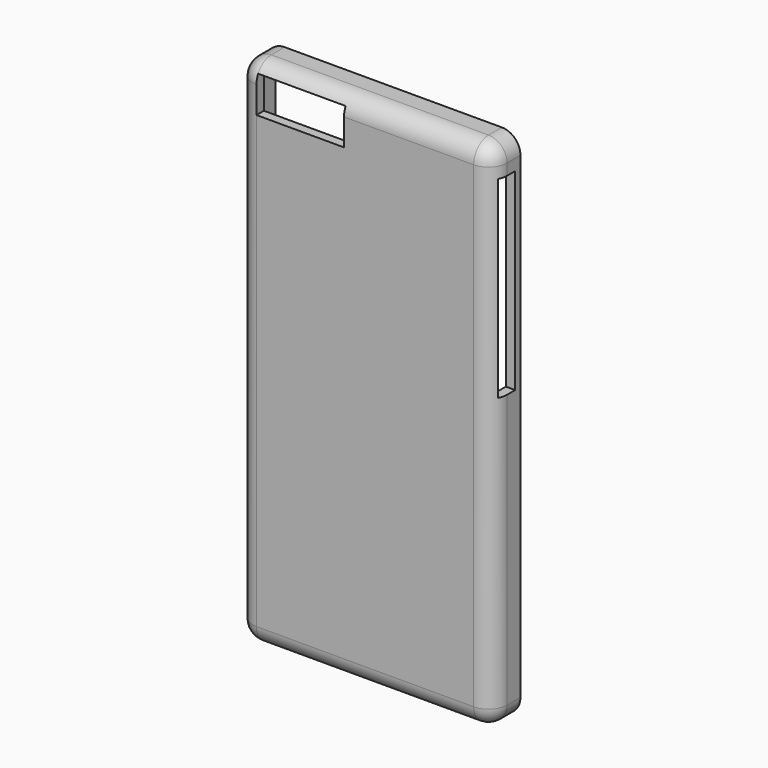
from build123d import *

# Parameters (mm, degrees)
F0_W        = 69.596
F0_H        = 140.716
F1_DEPTH    = 9.652
F2_R        = 5.08
F3_T1_DEPTH = 17.272
F3_S5_W     = 5.08
F3_S5_H     = 5.08
F3_T6_DEPTH = 5.08
F4_T1_DEPTH = 17.272
F4_S5_W     = 5.08
F4_S5_H     = 5.08
F4_T6_DEPTH = 5.08
F5_T1_DEPTH = 17.272
F5_S5_W     = 5.08
F5_S5_H     = 5.08
F5_T6_DEPTH = 5.08
F6_T        = -2.54
F7_W        = 23.9500291884
F7_H        = 9.7231566906
F8_DEPTH    = 25.4
F9_W        = 5.1087748725
F9_H        = 52.7357356623
F10_DEPTH   = 25.4
F11_W       = 4.6143759973
F11_H       = 14.0079259872
F12_DEPTH   = 25.4
F14_W       = 56.6909182817
F14_H       = 3.6255817395
F15_DEPTH   = 25.4


# Not quite as in the source:
# - a fillet or chamfer that OpenCascade refuses, or shapes differently, is made with other operations: its cross-section is extruded or revolved along the edge and cut away or added


with BuildPart() as f1:
    # F0 (on Front) → F1 (new body)
    with BuildSketch(Plane.XZ):
        Rectangle(F0_W, F0_H)
    extrude(amount=F1_DEPTH)

    # F2
    f2_edges = [f1.edges().sort_by_distance(p)[0] for p in [
        (-34.798, -4.826, 70.358),
        (0, -9.652, 70.358),
        (-34.798, -9.652, 0),
        (0, -9.652, -70.358),
        (34.798, -9.652, 0),
    ]]
    fillet(f2_edges, radius=F2_R)

    # F3: fillet of radius 5.08 on 1 edges, made by hand

    # F3_s2 → F3_t1 (cut)
    with BuildSketch(Plane.XZ.offset(-12.7)):
        with BuildLine():
            ThreePointArc((29.718, 70.358), (33.3101024484, 68.8701024484), (34.798, 65.278))
            Line((34.798, 65.278), (34.798, 70.358))
            Line((34.798, 70.358), (29.718, 70.358))
        make_face()
    extrude(amount=F3_T1_DEPTH, mode=Mode.SUBTRACT)


with BuildPart() as f3_tool4:
    # F3_s5 → F3_t6 (new body)
    with BuildSketch(Plane.XY.offset(65.278)):
        with Locations((32.258, -7.112)):
            Rectangle(F3_S5_W, F3_S5_H)
    extrude(amount=F3_T6_DEPTH)

    # F3_s7 → F3_t8 (revolve, cut)
    with BuildSketch(Plane(origin=(29.718, -4.572, 65.278), x_dir=(-0.7071067812, 0.7071067812, 0), z_dir=(0.7071067812, 0.7071067812, 0))):
        with BuildLine():
            ThreePointArc((0, -5.08), (5.08, 0), (0, 5.08))
            Line((0, 5.08), (0, -5.08))
        make_face()
    revolve(axis=Axis((29.718, -4.572, 65.278), (0, 0, 1)), mode=Mode.SUBTRACT)


with BuildPart() as f1_1:
    add(f1.part)

    # F3_t3: cut F3_tool4
    add(f3_tool4.part, mode=Mode.SUBTRACT)

    # F4: fillet of radius 5.08 on 1 edges, made by hand

    # F4_s2 → F4_t1 (cut)
    with BuildSketch(Plane.XZ.offset(-12.7)):
        with BuildLine():
            ThreePointArc((-29.718, -70.358), (-33.3101024484, -68.8701024484), (-34.798, -65.278))
            Line((-34.798, -65.278), (-34.798, -70.358))
            Line((-34.798, -70.358), (-29.718, -70.358))
        make_face()
    extrude(amount=F4_T1_DEPTH, mode=Mode.SUBTRACT)


with BuildPart() as f4_tool4:
    # F4_s5 → F4_t6 (new body)
    with BuildSketch(Plane.XY.offset(-65.278)):
        with Locations((-32.258, -7.112)):
            Rectangle(F4_S5_W, F4_S5_H)
    extrude(amount=-F4_T6_DEPTH)

    # F4_s7 → F4_t8 (revolve, cut)
    with BuildSketch(Plane(origin=(-29.718, -4.572, -65.278), x_dir=(0.7071067812, 0.7071067812, 0), z_dir=(-0.7071067812, 0.7071067812, 0))):
        with BuildLine():
            ThreePointArc((0, -5.08), (5.08, 0), (0, 5.08))
            Line((0, 5.08), (0, -5.08))
        make_face()
    revolve(axis=Axis((-29.718, -4.572, -65.278), (0, 0, -1)), mode=Mode.SUBTRACT)


with BuildPart() as f1_2:
    add(f1_1.part)

    # F4_t3: cut F4_tool4
    add(f4_tool4.part, mode=Mode.SUBTRACT)

    # F5: fillet of radius 5.08 on 1 edges, made by hand

    # F5_s2 → F5_t1 (cut)
    with BuildSketch(Plane.XZ.offset(-12.7)):
        with BuildLine():
            ThreePointArc((34.798, -65.278), (33.3101024484, -68.8701024484), (29.718, -70.358))
            Line((29.718, -70.358), (34.798, -70.358))
            Line((34.798, -70.358), (34.798, -65.278))
        make_face()
    extrude(amount=F5_T1_DEPTH, mode=Mode.SUBTRACT)


with BuildPart() as f5_tool4:
    # F5_s5 → F5_t6 (new body)
    with BuildSketch(Plane.YZ.offset(29.718)):
        with Locations((-7.112, -67.818)):
            Rectangle(F5_S5_W, F5_S5_H)
    extrude(amount=F5_T6_DEPTH)

    # F5_s7 → F5_t8 (revolve, cut)
    with BuildSketch(Plane(origin=(29.718, -4.572, -65.278), x_dir=(0, 0.7071067812, 0.7071067812), z_dir=(0, 0.7071067812, -0.7071067812))):
        with BuildLine():
            ThreePointArc((0, -5.08), (5.08, 0), (0, 5.08))
            Line((0, 5.08), (0, -5.08))
        make_face()
    revolve(axis=Axis((29.718, -4.572, -65.278), (1, 0, 0)), mode=Mode.SUBTRACT)


with BuildPart() as f1_3:
    add(f1_2.part)

    # F5_t3: cut F5_tool4
    add(f5_tool4.part, mode=Mode.SUBTRACT)

    # F6
    f6_openings = [f1_3.faces().sort_by_distance(p)[0] for p in [
        (0, 0, 0),
    ]]
    offset(amount=F6_T, openings=f6_openings)

    # F7 (on face) → F8 (cut)
    with BuildSketch(Plane.XZ.offset(9.652)):
        with Locations((-17.7429854058, 62.7884864807)):
            Rectangle(F7_W, F7_H)
    extrude(amount=-F8_DEPTH, mode=Mode.SUBTRACT)

    # F9 (on face) → F10 (cut)
    with BuildSketch(Plane.YZ.offset(34.798)):
        with Locations((-4.3671781896, 35.8438207768)):
            Rectangle(F9_W, F9_H)
    extrude(amount=-F10_DEPTH, mode=Mode.SUBTRACT)

    # F11 (on face) → F12 (cut)
    with BuildSketch(Plane(origin=(-34.798, 0, 0), x_dir=(0, -1, 0), z_dir=(-1, 0, 0))):
        with Locations((4.6143762302, 42.0237891376)):
            Rectangle(F11_W, F11_H)
    extrude(amount=-F12_DEPTH, mode=Mode.SUBTRACT)

    # F14 (on face) → F15 (cut)
    with BuildSketch(Plane(origin=(0, 0, -70.358), x_dir=(1, 0, 0), z_dir=(0, 0, -1))):
        with Locations((-0.3109676763, 3.6884165602)):
            Rectangle(F14_W, F14_H)
    extrude(amount=-F15_DEPTH, mode=Mode.SUBTRACT)


solid = f1_3.part
